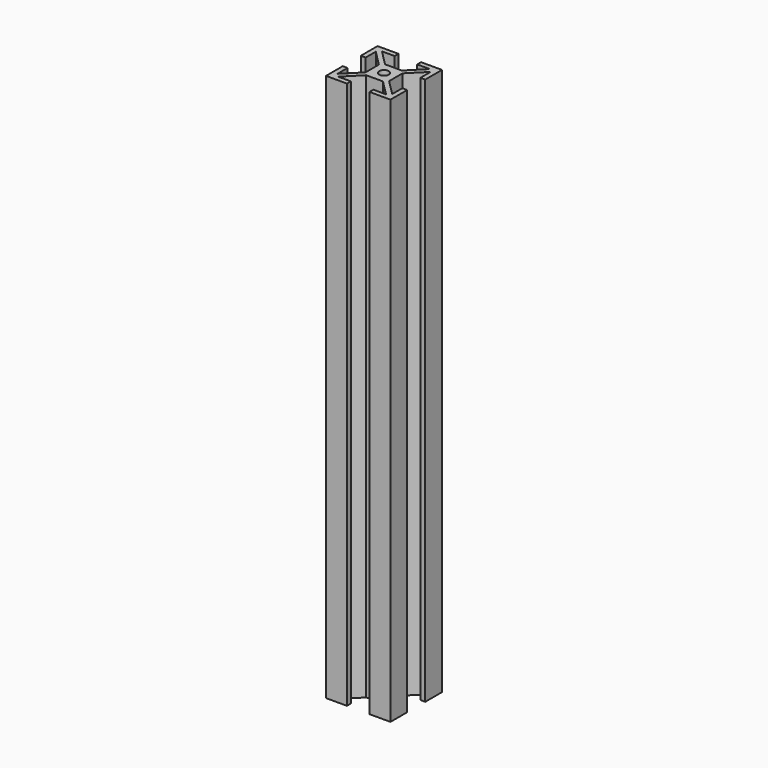
from build123d import *

# Parameters (mm, degrees)
F0_R            = 1.5
F1_DEPTH        = 170
F1_COPIES_COUNT = 4


# Not quite as in the source:
# - a pattern or mirror of a feature is missing from the dataset's text; its kind, count and spacing are read off the source's solid
# - a feature names something its author has since deleted; it is built from what else it names


with BuildPart() as f1:
    # F0 (on Top) → F1 (new body)
    with BuildSketch(Plane.XY):
        Polygon((-3.66, -3.66), (3.66, -3.66), (3.66, 3.66), (-2.5993398282, 3.66), (-3.66, 2.5993398282), align=None)
        Circle(F0_R, mode=Mode.SUBTRACT)
        Polygon((-8.5, 7.4393398282), (-3.66, 2.5993398282), (-2.5993398282, 3.66), (-7.4393398282, 8.5), (-3.5, 8.5), (-3.5, 10), (-10, 10), (-10, 3.5), (-8.5, 3.5), align=None)
    extrude(amount=F1_DEPTH)

    # F1_copies: F1 ×4 about axis
    f1_copies_axis = Axis((0, 0, 0), (0, 0, 1))


with BuildPart() as f1_1:
    add(f1.part)
    for i in range(1, F1_COPIES_COUNT):
        add(f1.part.rotate(f1_copies_axis, i * 360 / F1_COPIES_COUNT))


solid = f1_1.part
